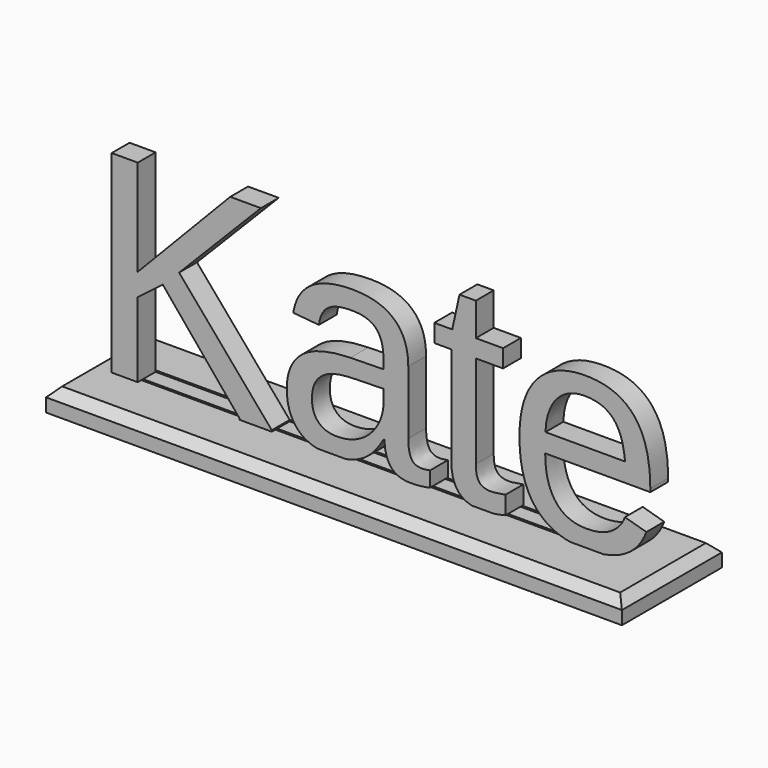
from build123d import *

# Parameters (mm, degrees)
F0_TEXT_SIZE = 158.75
F1_DEPTH     = 12.7
F2_W         = 14.8083984375
F2_H         = 12.7
F3_DEPTH     = 0.762
F4_W         = 18.3802734375
F4_H         = 12.7
F5_DEPTH     = 1.27
F6_W         = 8.89
F6_H         = 12.6975949547
F7_DEPTH     = 274.32
F8_W         = 327.66
F8_H         = 71.12
F8_W_2       = 276.86
F8_H_2       = 11.43
F9_DEPTH     = 12.7
F10_SIZE     = 5.08


# Not quite as in the source:
# - Text() gives the source's letters only with a copy of the font that has no kerning and outlines rounded to 1/6400 em; it was checked with that copy


with BuildPart() as f1:
    # F0 (on Front) → F1 (new body)
    with BuildSketch(Plane.XZ):
        with Locations((0, 0)):
            Text('Kate', F0_TEXT_SIZE, font='Arimo', text_align=(TextAlign.LEFT, TextAlign.BOTTOM))
    extrude(amount=F1_DEPTH)

    # F2 (on face) → F3 (join)
    with BuildSketch(Plane(origin=(0, 0, 0), x_dir=(1, 0, 0), z_dir=(0, 0, -1))):
        with Locations((20.4266601563, 6.35)):
            Rectangle(F2_W, F2_H)
    extrude(amount=F3_DEPTH)

    # F4 (on face) → F5 (join)
    with BuildSketch(Plane(origin=(0, 0, 0), x_dir=(1, 0, 0), z_dir=(0, 0, -1))):
        with Locations((94.9151367188, 6.35)):
            Rectangle(F4_W, F4_H)
    extrude(amount=F5_DEPTH)

    # F6 (on face) → F7 (join)
    with BuildSketch(Plane(origin=(13.0224609375, 0, 0), x_dir=(0, -1, 0), z_dir=(-1, 0, 0))):
        with Locations((4.445, -7.1107974773)):
            Rectangle(F6_W, F6_H)
    extrude(amount=-F7_DEPTH)


with BuildPart() as f9:
    # F8 (on face) → F9 (new body)
    with BuildSketch(Plane(origin=(0, 0, -13.4595949547), x_dir=(1, 0, 0), z_dir=(0, 0, -1))):
        with Locations((162.8824609375, 6.35)):
            Rectangle(F8_W, F8_H)
        with Locations((150.1824609375, 4.445)):
            Rectangle(F8_W_2, F8_H_2, mode=Mode.SUBTRACT)
    extrude(amount=-F9_DEPTH)

    # F10
    f10_edges = [f9.edges().sort_by_distance(p)[0] for p in [
        (162.882461, -41.91, -0.759595),
        (326.712461, -6.35, -0.759595),
        (162.882461, 29.21, -0.759595),
        (-0.947539, -6.35, -0.759595),
    ]]
    chamfer(f10_edges, length=F10_SIZE)


solid = Compound([f1.part, f9.part])
